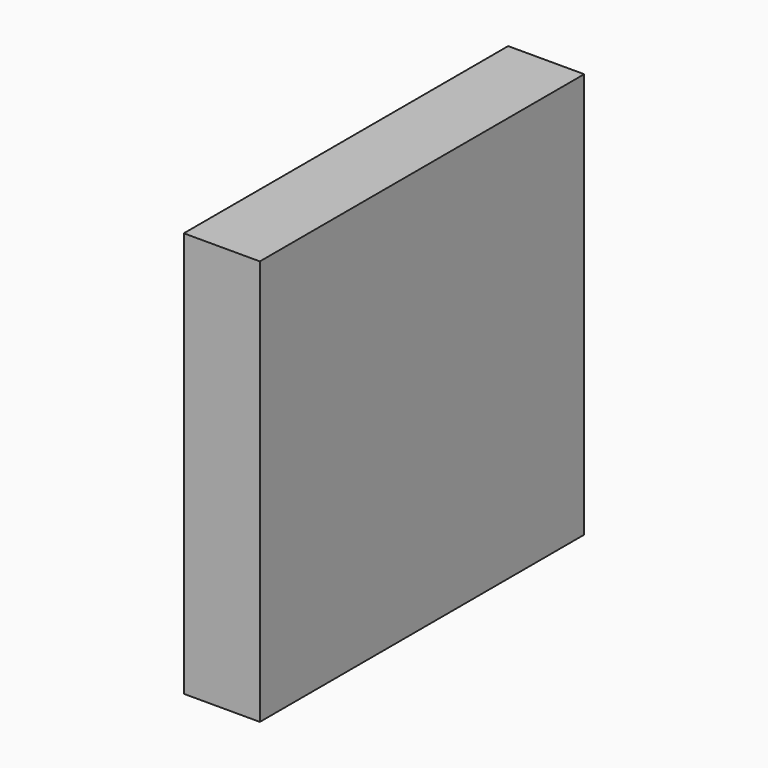
from build123d import *

# Parameters (mm, degrees)
F1_DEPTH = 10


# Not quite as in the source:
# - a feature names something its author has since deleted; it is built from what else it names


with BuildPart() as f1:
    # F0 (on Right) → F1 (new body)
    with BuildSketch(Plane.YZ):
        Polygon((22.5, 37.9), (0, 37.9), (-15.4, 37.9), (-15.4, 15), (-15.4, 7.5), (-15.4, -15.4), (0, -15.4), (22.5, -15.4), (37.9, -15.4), (37.9, 0), (37.9, 22.5), (37.9, 37.9), align=None)
    extrude(amount=-F1_DEPTH)


solid = f1.part
